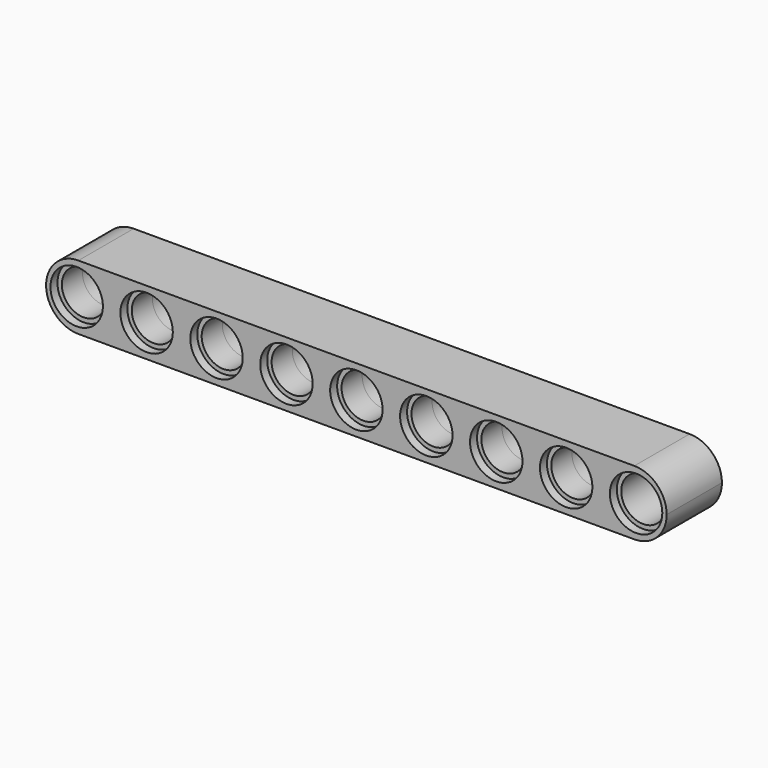
from build123d import *

# Parameters (mm, degrees)
F0_W     = 71
F0_H     = 7.4
F0_R     = 3
F1_DEPTH = 3.95
F0_R_2   = 2.499
F2_DEPTH = 2.95
F3_R     = 3.69999


# Not quite as in the source:
# - a fillet or chamfer is up to 0.001 mm smaller than in the source, because OpenCascade refuses the exact size


with BuildPart() as f1:
    # F0 (on Front) → F1 (new body, symmetric)
    with BuildSketch(Plane.XZ):
        Rectangle(F0_W, F0_H)
        with Locations((-32, 0)):
            Circle(F0_R, mode=Mode.SUBTRACT)
        with Locations((-24, 0)):
            Circle(F0_R, mode=Mode.SUBTRACT)
        with Locations((-16, 0)):
            Circle(F0_R, mode=Mode.SUBTRACT)
        with Locations((-8, 0)):
            Circle(F0_R, mode=Mode.SUBTRACT)
        Circle(F0_R, mode=Mode.SUBTRACT)
        with Locations((8, 0)):
            Circle(F0_R, mode=Mode.SUBTRACT)
        with Locations((16, 0)):
            Circle(F0_R, mode=Mode.SUBTRACT)
        with Locations((24, 0)):
            Circle(F0_R, mode=Mode.SUBTRACT)
        with Locations((32, 0)):
            Circle(F0_R, mode=Mode.SUBTRACT)
    extrude(amount=F1_DEPTH, both=True)

    # F0 (on Front) → F2 (join, symmetric)
    with BuildSketch(Plane.XZ):
        with Locations((-32, 0)):
            Circle(F0_R)
        with Locations((-32, 0)):
            Circle(F0_R_2, mode=Mode.SUBTRACT)
        with Locations((-24, 0)):
            Circle(F0_R)
        with Locations((-24, 0)):
            Circle(F0_R_2, mode=Mode.SUBTRACT)
        with Locations((-16, 0)):
            Circle(F0_R)
        with Locations((-16, 0)):
            Circle(F0_R_2, mode=Mode.SUBTRACT)
        with Locations((-8, 0)):
            Circle(F0_R)
        with Locations((-8, 0)):
            Circle(F0_R_2, mode=Mode.SUBTRACT)
        Circle(F0_R)
        Circle(F0_R_2, mode=Mode.SUBTRACT)
        with Locations((8, 0)):
            Circle(F0_R)
        with Locations((8, 0)):
            Circle(F0_R_2, mode=Mode.SUBTRACT)
        with Locations((16, 0)):
            Circle(F0_R)
        with Locations((16, 0)):
            Circle(F0_R_2, mode=Mode.SUBTRACT)
        with Locations((24, 0)):
            Circle(F0_R)
        with Locations((24, 0)):
            Circle(F0_R_2, mode=Mode.SUBTRACT)
        with Locations((32, 0)):
            Circle(F0_R)
        with Locations((32, 0)):
            Circle(F0_R_2, mode=Mode.SUBTRACT)
    extrude(amount=F2_DEPTH, both=True)

    # F3 (radius 3.7 in the source; OpenCascade refuses exactly that, so slightly less here)
    f3_edges = [f1.edges().sort_by_distance(p)[0] for p in [
        (-35.5, 0, 3.7),
        (-35.5, 0, -3.7),
        (35.5, 0, 3.7),
        (35.5, 0, -3.7),
    ]]
    fillet(f3_edges, radius=F3_R)


solid = f1.part
